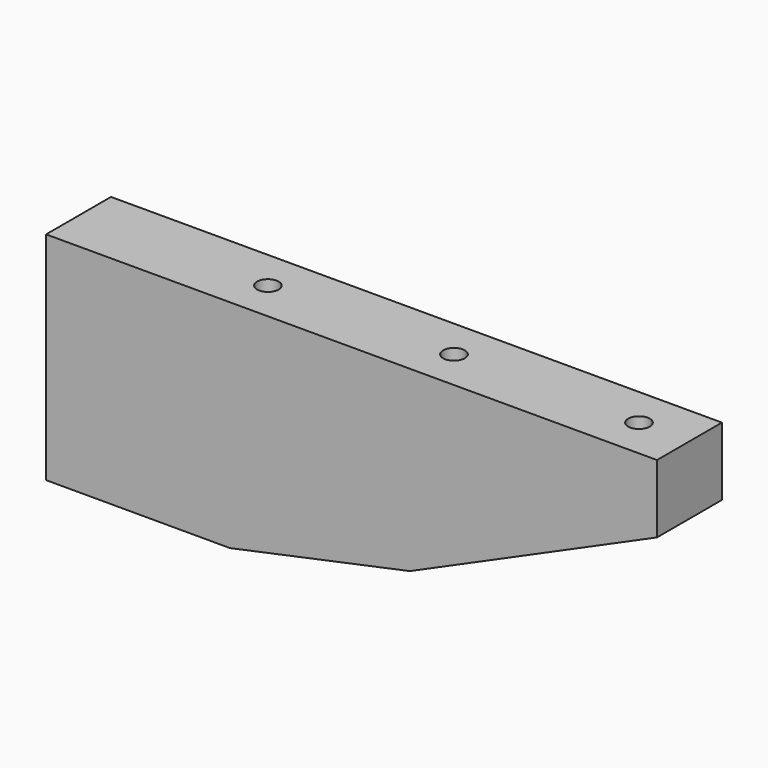
from build123d import *

# Parameters (mm, degrees)
F1_DEPTH  = 19.05
F2_R      = 2.54
F3_DEPTH  = 50.801
F4_START  = -13.97
F2_R_2    = 4.445
F4_DEPTH  = 40.386
F6_DEPTH  = 10.16
F8_DEPTH  = 10.16
F10_DEPTH = 10.16


with BuildPart() as f1:
    # F0 (on Front) → F1 (new body)
    with BuildSketch(Plane.XZ):
        Polygon((149.77654996, 57.15), (6.35, 57.15), (6.35, 6.35), (49.53, 6.35), (91.7664133997, 15.3276268095), (149.77654996, 41.1554036448), align=None)
    extrude(amount=F1_DEPTH)

    # F2 (on face) → F3 (cut, through all)
    with BuildSketch(Plane.XY.offset(57.15)):
        with Locations((50.8, -9.525)):
            Circle(F2_R)
        with Locations((94.488, -9.525)):
            Circle(F2_R)
        with Locations((137.922, -9.525)):
            Circle(F2_R)
    extrude(amount=-F3_DEPTH, mode=Mode.SUBTRACT)

    # F2 (on face) → F4 (cut)
    with BuildSketch(Plane.XY.offset(57.15).offset(F4_START)):
        with Locations((50.8, -9.525)):
            Circle(F2_R_2)
        with Locations((50.8, -9.525)):
            Circle(F2_R, mode=Mode.SUBTRACT)
        with Locations((94.488, -9.525)):
            Circle(F2_R_2)
        with Locations((94.488, -9.525)):
            Circle(F2_R, mode=Mode.SUBTRACT)
        with Locations((137.922, -9.525)):
            Circle(F2_R_2)
        with Locations((137.922, -9.525)):
            Circle(F2_R, mode=Mode.SUBTRACT)
    extrude(amount=-F4_DEPTH, mode=Mode.SUBTRACT)

    # F5 (on face) → F6 (cut)
    with BuildSketch(Plane(origin=(0, 0, 6.35), x_dir=(1, 0, 0), z_dir=(0, 0, -1))):
        with BuildLine():
            ThreePointArc((21.0968814449, 14.0652501177), (20.97463405, 14.5484294642), (20.6373100259, 14.915334369))
            ThreePointArc((20.6373100259, 14.915334369), (20.0808814449, 14.0652501177), (19.6229011784, 13.1583267056))
            ThreePointArc((19.6229011784, 13.1583267056), (20.6133042324, 13.1999282265), (21.0968814449, 14.0652501177))
        make_face()
        with BuildLine():
            ThreePointArc((19.6229011784, 13.1583267056), (20.0808814449, 14.0652501177), (20.6373100259, 14.915334369))
            ThreePointArc((20.6373100259, 14.915334369), (19.2009996347, 14.5732501177), (19.6229011784, 13.1583267056))
        make_face()
        with BuildLine():
            ThreePointArc((36.8247688031, 4.9847501177), (36.6740906943, 5.5171729052), (36.2667490696, 5.8916735299))
            ThreePointArc((36.2667490696, 5.8916735299), (35.8087688031, 4.9847501177), (35.2523402221, 4.1346658664))
            ThreePointArc((35.2523402221, 4.1346658664), (36.2919481496, 4.0909975126), (36.8247688031, 4.9847501177))
        make_face()
        with BuildLine():
            ThreePointArc((35.2523402221, 4.1346658664), (35.8087688031, 4.9847501177), (36.2667490696, 5.8916735299))
            ThreePointArc((36.2667490696, 5.8916735299), (34.9288869928, 5.4927501177), (35.2523402221, 4.1346658664))
        make_face()
    extrude(amount=-F6_DEPTH, mode=Mode.SUBTRACT)

    # F7 (on face) → F8 (cut)
    with BuildSketch(Plane(origin=(0.8496578997, 0, -3.9973261378), x_dir=(0.9781476007, 0, 0.2079116908), z_dir=(0.2079116908, 0, -0.9781476007))):
        with BuildLine():
            ThreePointArc((64.5139077337, 14.0652501177), (64.3916603388, 14.5484294642), (64.0543363147, 14.915334369))
            ThreePointArc((64.0543363147, 14.915334369), (63.4979077337, 14.0652501177), (63.0399274672, 13.1583267056))
            ThreePointArc((63.0399274672, 13.1583267056), (64.0303305212, 13.1999282265), (64.5139077337, 14.0652501177))
        make_face()
        with BuildLine():
            ThreePointArc((63.0399274672, 13.1583267056), (63.4979077337, 14.0652501177), (64.0543363147, 14.915334369))
            ThreePointArc((64.0543363147, 14.915334369), (62.6180259235, 14.5732501177), (63.0399274672, 13.1583267056))
        make_face()
        with BuildLine():
            ThreePointArc((80.2417950919, 4.9847501177), (80.0911169831, 5.5171729052), (79.6837753584, 5.8916735299))
            ThreePointArc((79.6837753584, 5.8916735299), (79.2257950919, 4.9847501177), (78.6693665109, 4.1346658664))
            ThreePointArc((78.6693665109, 4.1346658664), (79.7089744384, 4.0909975126), (80.2417950919, 4.9847501177))
        make_face()
        with BuildLine():
            ThreePointArc((78.6693665109, 4.1346658664), (79.2257950919, 4.9847501177), (79.6837753584, 5.8916735299))
            ThreePointArc((79.6837753584, 5.8916735299), (78.3459132816, 5.4927501177), (78.6693665109, 4.1346658664))
        make_face()
    extrude(amount=-F8_DEPTH, mode=Mode.SUBTRACT)

    # F9 (on face) → F10 (cut)
    with BuildSketch(Plane(origin=(9.4860255039, 0, -21.30596212), x_dir=(0.9135454576, 0, 0.4067366431), z_dir=(0.4067366431, 0, -0.9135454576))):
        with BuildLine():
            ThreePointArc((105.3219744595, 14.06525), (105.1997270646, 14.5484293465), (104.8624030404, 14.9153342513))
            ThreePointArc((104.8624030404, 14.9153342513), (104.3059744595, 14.06525), (103.847994193, 13.1583265879))
            ThreePointArc((103.847994193, 13.1583265879), (104.8383972469, 13.1999281088), (105.3219744595, 14.06525))
        make_face()
        with BuildLine():
            ThreePointArc((103.847994193, 13.1583265879), (104.3059744595, 14.06525), (104.8624030404, 14.9153342513))
            ThreePointArc((104.8624030404, 14.9153342513), (103.4260926492, 14.57325), (103.847994193, 13.1583265879))
        make_face()
        with BuildLine():
            ThreePointArc((121.0498618176, 4.98475), (120.8991837088, 5.5171727875), (120.4918420841, 5.8916734121))
            ThreePointArc((120.4918420841, 5.8916734121), (120.0338618176, 4.98475), (119.4774332367, 4.1346657487))
            ThreePointArc((119.4774332367, 4.1346657487), (120.5170411641, 4.0909973949), (121.0498618176, 4.98475))
        make_face()
        with BuildLine():
            ThreePointArc((119.4774332367, 4.1346657487), (120.0338618176, 4.98475), (120.4918420841, 5.8916734121))
            ThreePointArc((120.4918420841, 5.8916734121), (119.1539800074, 5.49275), (119.4774332367, 4.1346657487))
        make_face()
    extrude(amount=-F10_DEPTH, mode=Mode.SUBTRACT)


solid = f1.part
